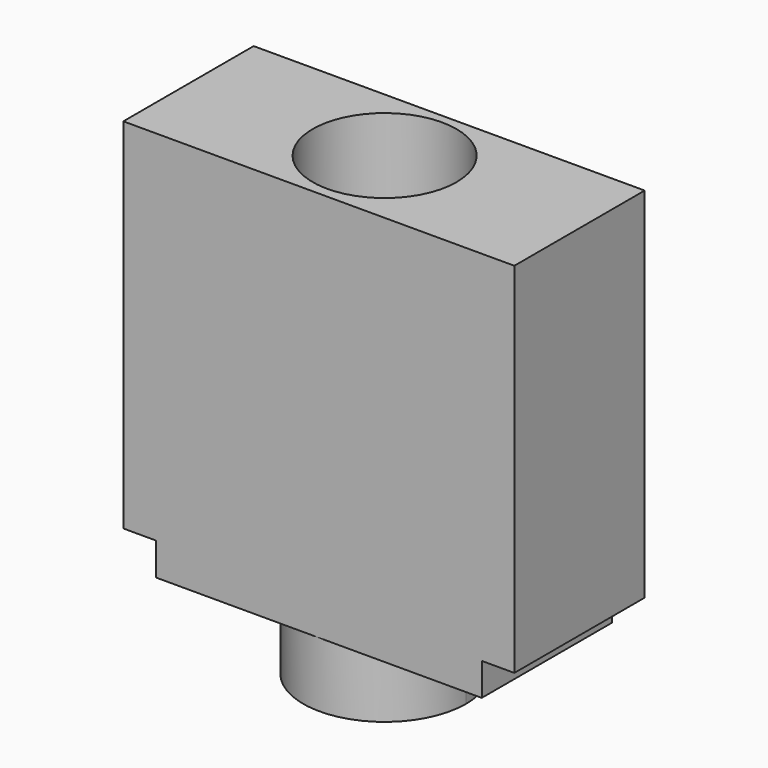
from build123d import *

# Parameters (mm, degrees)
F1_DEPTH = 5
F3_DEPTH = 2
F4_R     = 2.20671025
F5_DEPTH = 25


with BuildPart() as f1:
    # F0 (on Front) → F1 (new body)
    with BuildSketch(Plane.XZ):
        Polygon((0, 11), (-12, 11), (-12, 0), (-11, 0), (-11, -1), (-1, -1), (-1, 0), (0, 0), align=None)
    extrude(amount=F1_DEPTH)

    # F2 (on face) → F3 (join)
    with BuildSketch(Plane(origin=(0, 0, -1), x_dir=(1, 0, 0), z_dir=(0, 0, -1))):
        with BuildLine():
            ThreePointArc((-5.6578661307, 0), (-4.1151479271, 0.8341224011), (-3.5, 2.4764782283))
            ThreePointArc((-3.5, 2.4764782283), (-7.6423558273, 4.3613303012), (-6.3421338693, 0))
            Line((-6.3421338693, 0), (-5.6578661307, 0))
        make_face()
    extrude(amount=F3_DEPTH)

    # F4 (on face) → F5 (cut)
    with BuildSketch(Plane(origin=(0, 0, -3), x_dir=(1, 0, 0), z_dir=(0, 0, -1))):
        with Locations((-6, 2.4764782283)):
            Circle(F4_R)
    extrude(amount=-F5_DEPTH, mode=Mode.SUBTRACT)


solid = f1.part
